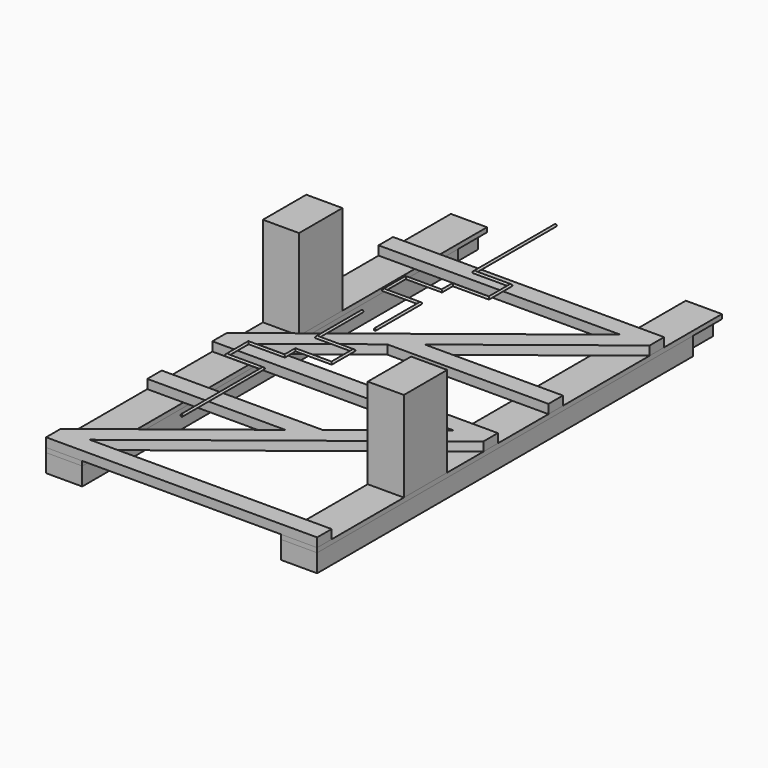
from build123d import *

# Parameters (mm, degrees)
F2_START = -25.4
F1_W     = 203.2
F1_H     = 304.8
F1_H_2   = 1524
F2_DEPTH = 101.6
F1_H_3   = 609.6
F3_DEPTH = 508
F4_DEPTH = 508
F1_W_2   = 50.8
F1_H_4   = 203.2
F6_DEPTH = 25.4
F7_W     = 558.8
F7_H     = 101.6
F7_W_2   = 203.2
F8_DEPTH = 50.8
F12_R    = 6.35
F14_R    = 6.35


with BuildPart() as f2:
    # F1 (on Top) → F2 (new body)
    with BuildSketch(Plane.XY.offset(F2_START)):
        Polygon((-762, 1422.4), (-762, 1219.2), (-660.4, 1219.2), (-660.4, 1422.4), (-711.2, 1422.4), align=None)
        Polygon((-660.4, 1219.2), (-762, 1219.2), (-762, 609.6), (-558.8, 609.6), (-558.8, 1219.2), align=None)
        Polygon((-660.4, 1422.4), (-660.4, 1219.2), (-558.8, 1219.2), (-558.8, 1422.4), (-609.6, 1422.4), align=None)
        with Locations((-660.4, 457.2)):
            Rectangle(F1_W, F1_H)
        Polygon((-711.2, 1422.4), (-660.4, 1422.4), (-609.6, 1422.4), (-609.6, 1625.6), (-711.2, 1625.6), align=None)
        with Locations((-660.4, -457.2)):
            Rectangle(F1_W, F1_H_2)
        Polygon((-660.4, 1651), (-711.2, 1625.6), (-609.6, 1625.6), align=None)
    extrude(amount=-F2_DEPTH)


with BuildPart() as f2b:
    # F1 (on Top) → F2, piece 2 (new body)
    with BuildSketch(Plane.XY.offset(F2_START)):
        Polygon((660.4, 1219.2), (558.8, 1219.2), (558.8, -304.8), (762, -304.8), (762, 1219.2), align=None)
        Polygon((558.8, 1422.4), (558.8, 1219.2), (660.4, 1219.2), (660.4, 1422.4), (609.6, 1422.4), align=None)
        with Locations((660.4, -457.2)):
            Rectangle(F1_W, F1_H)
        Polygon((660.4, 1422.4), (660.4, 1219.2), (762, 1219.2), (762, 1422.4), (711.2, 1422.4), align=None)
        with Locations((660.4, -914.4)):
            Rectangle(F1_W, F1_H_3)
        Polygon((609.6, 1422.4), (660.4, 1422.4), (711.2, 1422.4), (711.2, 1625.6), (609.6, 1625.6), align=None)
    extrude(amount=-F2_DEPTH)


with BuildPart() as f3:
    # F1 (on Top) → F3 (new body)
    with BuildSketch(Plane.XY):
        with Locations((-660.4, 457.2)):
            Rectangle(F1_W, F1_H)
    extrude(amount=F3_DEPTH)


with BuildPart() as f4:
    # F1 (on Top) → F4 (new body)
    with BuildSketch(Plane.XY):
        with Locations((660.4, -457.2)):
            Rectangle(F1_W, F1_H)
    extrude(amount=F4_DEPTH)


with BuildPart() as f6:
    # F1 (on Top) → F6 (new body)
    with BuildSketch(Plane.XY):
        with Locations((-736.6, 1524)):
            Rectangle(F1_W_2, F1_H_4)
        Polygon((-711.2, 1422.4), (-660.4, 1422.4), (-609.6, 1422.4), (-609.6, 1625.6), (-711.2, 1625.6), align=None)
        with Locations((-584.2, 1524)):
            Rectangle(F1_W_2, F1_H_4)
        Polygon((-660.4, 1422.4), (-660.4, 1219.2), (-558.8, 1219.2), (-558.8, 1422.4), (-609.6, 1422.4), align=None)
        Polygon((-762, 1422.4), (-762, 1219.2), (-660.4, 1219.2), (-660.4, 1422.4), (-711.2, 1422.4), align=None)
        Polygon((-660.4, 1219.2), (-762, 1219.2), (-762, 609.6), (-558.8, 609.6), (-558.8, 1219.2), align=None)
        with Locations((-660.4, -457.2)):
            Rectangle(F1_W, F1_H_2)
        with Locations((-660.4, 457.2)):
            Rectangle(F1_W, F1_H)
    extrude(amount=-F6_DEPTH)


with BuildPart() as f6b:
    # F1 (on Top) → F6, piece 2 (new body)
    with BuildSketch(Plane.XY):
        Polygon((660.4, 1219.2), (558.8, 1219.2), (558.8, -304.8), (762, -304.8), (762, 1219.2), align=None)
        with Locations((660.4, -914.4)):
            Rectangle(F1_W, F1_H_3)
        with Locations((584.2, 1524)):
            Rectangle(F1_W_2, F1_H_4)
        Polygon((609.6, 1422.4), (660.4, 1422.4), (711.2, 1422.4), (711.2, 1625.6), (609.6, 1625.6), align=None)
        with Locations((736.6, 1524)):
            Rectangle(F1_W_2, F1_H_4)
        Polygon((660.4, 1422.4), (660.4, 1219.2), (762, 1219.2), (762, 1422.4), (711.2, 1422.4), align=None)
        Polygon((558.8, 1422.4), (558.8, 1219.2), (660.4, 1219.2), (660.4, 1422.4), (609.6, 1422.4), align=None)
        with Locations((660.4, -457.2)):
            Rectangle(F1_W, F1_H)
    extrude(amount=-F6_DEPTH)


with BuildPart() as f8:
    # F7 (on Top) → F8 (new body)
    with BuildSketch(Plane.XY):
        Polygon((0, 648.7744153468), (-558.8, 210.2598440925), (-558.8, 81.111013399), (-144.2835902197, 406.4), (-14.8145059026, 508), (0, 519.6255846532), align=None)
        Polygon((-558.8, 210.2598440925), (-762, 50.8), (-597.4253853296, 50.8), (-558.8, 81.111013399), align=None)
        Polygon((558.8, 1087.288986601), (0, 648.7744153468), (0, 519.6255846532), (558.8, 958.1401559075), align=None)
        Polygon((597.4253853296, 1117.6), (558.8, 1087.288986601), (558.8, 958.1401559075), (762, 1117.6), align=None)
        Polygon((762, 1219.2), (558.8, 1219.2), (558.8, 1117.6), (597.4253853296, 1117.6), (762, 1117.6), align=None)
        with Locations((279.4, 1168.4)):
            Rectangle(F7_W, F7_H)
        with Locations((-279.4, 1168.4)):
            Rectangle(F7_W, F7_H)
        with Locations((-660.4, 1168.4)):
            Rectangle(F7_W_2, F7_H)
        with Locations((-279.4, 0)):
            Rectangle(F7_W, F7_H)
        Polygon((-597.4253853296, 50.8), (-762, 50.8), (-762, -50.8), (-558.8, -50.8), (-558.8, 50.8), align=None)
        with Locations((279.4, 0)):
            Rectangle(F7_W, F7_H)
        Polygon((558.8, 50.8), (558.8, -50.8), (597.4253853296, -50.8), (762, -50.8), (762, 50.8), align=None)
        Polygon((558.8, -81.111013399), (144.2835902197, -406.4), (14.8145059026, -508), (0, -519.6255846533), (0, -648.7744153467), (558.8, -210.2598440925), align=None)
        Polygon((597.4253853296, -50.8), (558.8, -81.111013399), (558.8, -210.2598440925), (762, -50.8), align=None)
        Polygon((0, -519.6255846533), (-558.8, -958.1401559075), (-558.8, -1087.288986601), (0, -648.7744153467), align=None)
        Polygon((-558.8, -958.1401559075), (-762, -1117.6), (-597.4253853296, -1117.6), (-558.8, -1087.288986601), align=None)
        with Locations((-279.4, -1168.4)):
            Rectangle(F7_W, F7_H)
        Polygon((-597.4253853296, -1117.6), (-762, -1117.6), (-762, -1219.2), (-558.8, -1219.2), (-558.8, -1117.6), align=None)
        with Locations((279.4, -1168.4)):
            Rectangle(F7_W, F7_H)
        with Locations((660.4, -1168.4)):
            Rectangle(F7_W_2, F7_H)
        with Locations((-279.4, -457.2)):
            Rectangle(F7_W, F7_H)
        with Locations((-660.4, -457.2)):
            Rectangle(F7_W_2, F7_H)
        Polygon((144.2835902197, -406.4), (0, -406.4), (0, -508), (14.8145059026, -508), align=None)
        Polygon((-14.8145059026, 508), (-144.2835902197, 406.4), (0, 406.4), (0, 508), align=None)
        with Locations((660.4, 457.2)):
            Rectangle(F7_W_2, F7_H)
        with Locations((279.4, 457.2)):
            Rectangle(F7_W, F7_H)
    extrude(amount=F8_DEPTH)


with BuildPart() as f13:
    # F13: sweep along a path in F5
    with BuildLine(Plane.XY.offset(406.4)) as f13_path:
        Line((152.4, 1219.2), (152.4, 647.7))
        Line((152.4, 647.7), (355.6, 647.7))
        Line((355.6, 647.7), (355.6, 495.3))
        Line((355.6, 495.3), (152.4, 495.3))
        Line((152.4, 495.3), (152.4, 419.1))
        Line((152.4, 419.1), (-50.8, 419.1))
        Line((-50.8, 419.1), (-50.8, 266.7))
        Line((-50.8, 266.7), (152.4, 266.7))
        Line((152.4, 266.7), (152.4, -50.8))
    # F12 (on offset) → F13 (sweep)
    with BuildSketch(Plane(origin=(0, 1219.2, 0), x_dir=(-1, 0, 0), z_dir=(0, 1, 0))):
        with Locations((-152.4, 406.4)):
            Circle(F12_R)
    sweep(path=f13_path.line, transition=Transition.RIGHT)


with BuildPart() as f15:
    # F15: sweep along a path in F5
    with BuildLine(Plane.XY.offset(406.4)) as f15_path:
        Line((0, -1219.2), (0, -647.7))
        Line((0, -647.7), (-203.2, -647.7))
        Line((-203.2, -647.7), (-203.2, -495.3))
        Line((-203.2, -495.3), (0, -495.3))
        Line((0, -495.3), (0, -419.1))
        Line((0, -419.1), (203.2, -419.1))
        Line((203.2, -419.1), (203.2, -266.7))
        Line((203.2, -266.7), (0, -266.7))
        Line((0, -266.7), (0, 50.8))
    # F14 (on offset) → F15 (sweep)
    with BuildSketch(Plane.XZ.offset(1219.2)):
        with Locations((0, 406.4)):
            Circle(F14_R)
    sweep(path=f15_path.line, transition=Transition.RIGHT)


solid = Compound([f2.part, f2b.part, f3.part, f4.part, f6.part, f6b.part, f8.part, f13.part, f15.part])
